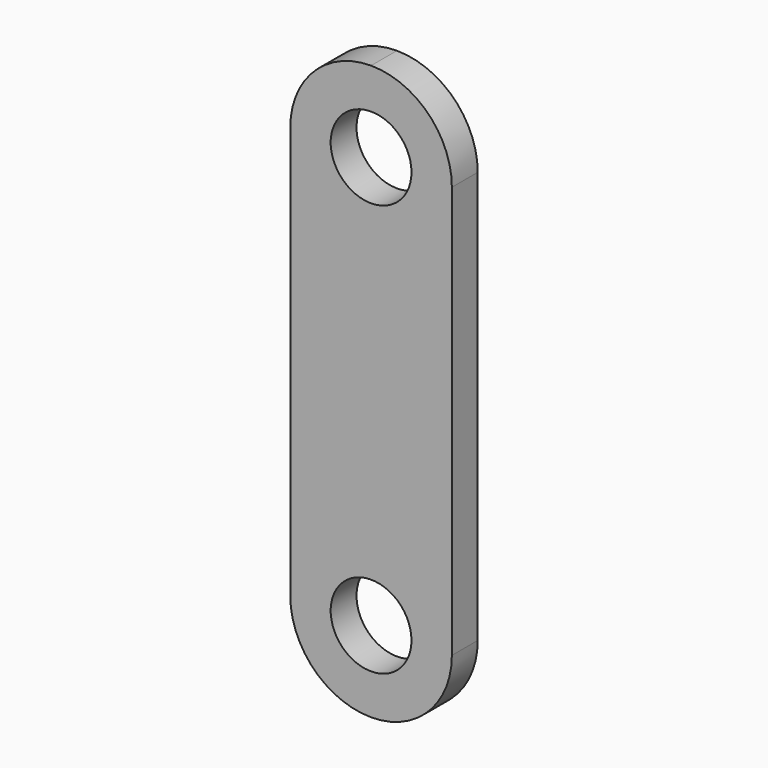
from build123d import *

# Parameters (mm, degrees)
F0_W     = 100
F0_H     = 355
F0_R     = 25
F1_DEPTH = 20
F2_R     = 49.99999


# Not quite as in the source:
# - a fillet or chamfer is up to 0.001 mm smaller than in the source, because OpenCascade refuses the exact size


with BuildPart() as f1:
    # F0 (on Front) → F1 (new body)
    with BuildSketch(Plane.XZ):
        Rectangle(F0_W, F0_H)
        with Locations((0, -127.5)):
            Circle(F0_R, mode=Mode.SUBTRACT)
        with Locations((0, 127.5)):
            Circle(F0_R, mode=Mode.SUBTRACT)
    extrude(amount=F1_DEPTH)

    # F2 (radius 50 in the source; OpenCascade refuses exactly that, so slightly less here)
    f2_edges = [f1.edges().sort_by_distance(p)[0] for p in [
        (50, -10, 177.5),
        (-50, -10, 177.5),
        (50, -10, -177.5),
        (-50, -10, -177.5),
    ]]
    fillet(f2_edges, radius=F2_R)


solid = f1.part
